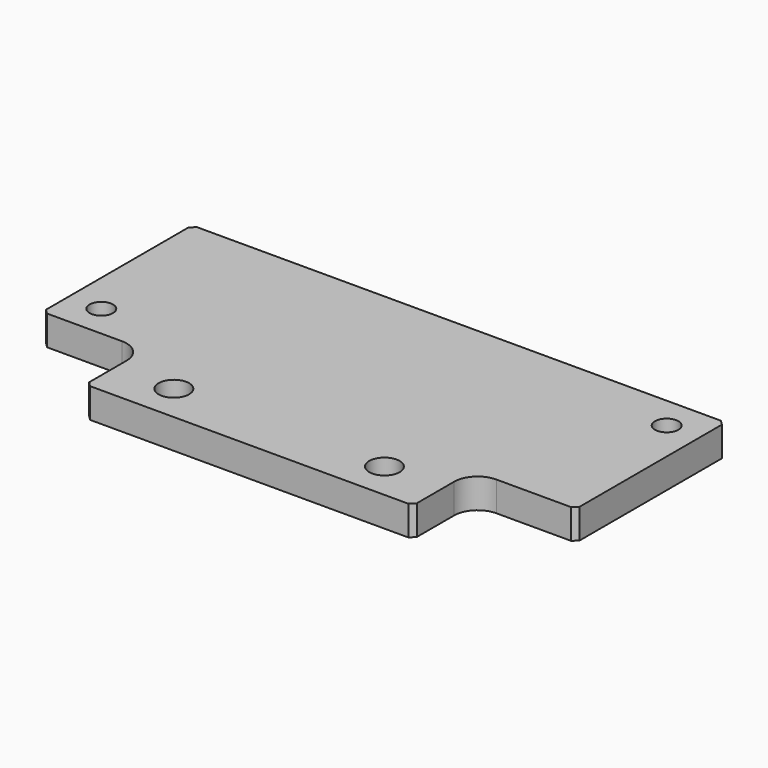
from build123d import *

# Parameters (mm, degrees)
F0_R     = 3.25
F1_DEPTH = 6.35
F2_SIZE  = 1
F3_D     = 5


with BuildPart() as f1:
    # F0 (on Top) → F1 (new body)
    with BuildSketch(Plane.XY):
        with BuildLine():
            Line((57, -20), (57, 20))
            Line((57, 20), (-57, 20))
            Line((-57, 20), (-57, -20))
            Line((-57, -20), (-40, -20))
            ThreePointArc((-40, -20), (-36.4644660941, -21.4644660941), (-35, -25))
            Line((-35, -25), (-35, -36))
            Line((-35, -36), (35, -36))
            Line((35, -36), (35, -25))
            ThreePointArc((35, -25), (36.4644660941, -21.4644660941), (40, -20))
            Line((40, -20), (57, -20))
        make_face()
        with Locations((-22.5, -28)):
            Circle(F0_R, mode=Mode.SUBTRACT)
        with Locations((22.5, -28)):
            Circle(F0_R, mode=Mode.SUBTRACT)
    extrude(amount=-F1_DEPTH)

    # F2
    f2_edges = [f1.edges().sort_by_distance(p)[0] for p in [
        (-35, -36, -3.175),
        (-57, -20, -3.175),
        (35, -36, -3.175),
        (57, -20, -3.175),
        (-57, 20, -3.175),
        (57, 20, -3.175),
    ]]
    chamfer(f2_edges, length=F2_SIZE)

    # F3 (through all)
    with Locations(Plane.XY):
        with Locations((-50, -13), (50, 13)):
            Hole(F3_D / 2)


solid = f1.part
